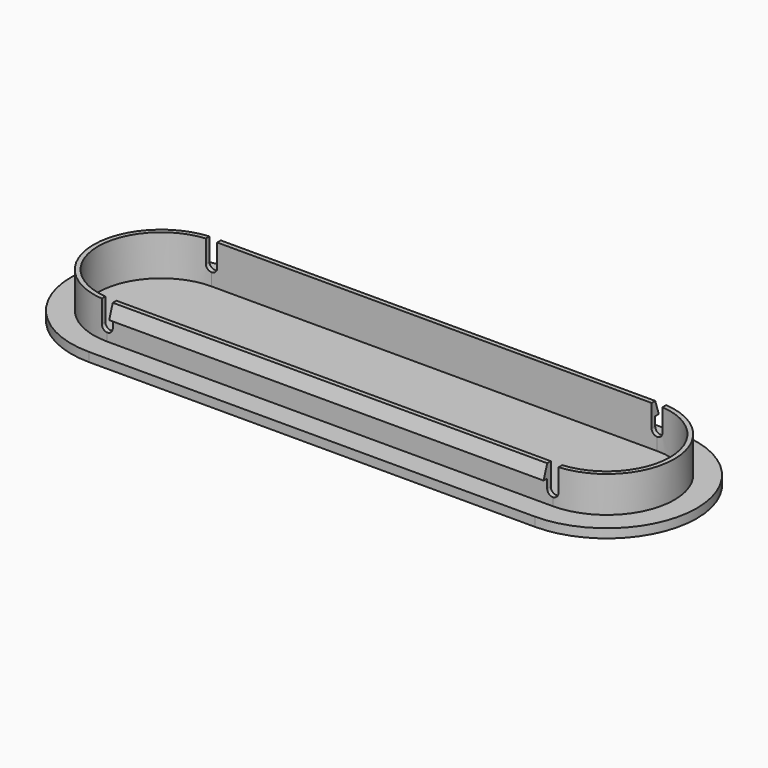
from build123d import *

# Parameters (mm, degrees)
F1_DEPTH      = 2
F2_DEPTH      = 8
F3_T          = 1
F3_T3_DEPTH   = 101
F3_T6_ANGLE   = 180.000000001
F3_T8_ANGLE   = 180.000000001
F7_DEPTH      = 25
F7_DEPTH_BACK = 25


# Not quite as in the source:
# - a shell that OpenCascade refuses in one call is made with other operations: the cavity is built on its own and cut out


with BuildPart() as f1:
    # F0 (on Top) → F1 (new body)
    with BuildSketch(Plane.XY):
        with BuildLine():
            Line((0, 19.999999553), (-99, 19.999999553))
            ThreePointArc((-99, 19.999999553), (-118.999999553, 0), (-99, -19.999999553))
            Line((-99, -19.999999553), (0, -19.999999553))
            ThreePointArc((0, -19.999999553), (19.999999553, 0), (0, 19.999999553))
        make_face()
        with BuildLine():
            ThreePointArc((0, 15), (15, 0), (0, -15))
            Line((0, -15), (-99, -15))
            ThreePointArc((-99, -15), (-114, 0), (-99, 15))
            Line((-99, 15), (0, 15))
        make_face(mode=Mode.SUBTRACT)
        with BuildLine():
            Line((-99, -15), (0, -15))
            ThreePointArc((0, -15), (15, 0), (0, 15))
            Line((0, 15), (-99, 15))
            ThreePointArc((-99, 15), (-114, 0), (-99, -15))
        make_face()
    extrude(amount=-F1_DEPTH)

    # F0 (on Top) → F2 (join)
    with BuildSketch(Plane.XY):
        with BuildLine():
            Line((-99, -15), (0, -15))
            ThreePointArc((0, -15), (15, 0), (0, 15))
            Line((0, 15), (-99, 15))
            ThreePointArc((-99, 15), (-114, 0), (-99, -15))
        make_face()
    extrude(amount=F2_DEPTH)

    # F3: shell of thickness 1, made by hand


with BuildPart() as f3_core1:
    # F3_t2: copy of F1
    add(f1.part)

    # the walls: a layer under each face that stays
    f3_faces = [f3_core1.faces().sort_by_distance(p)[0] for p in [
        (-49.5, -19.999999553, -1),
        (-118.999999553, 0, -1),
        (19.999999553, 0, -1),
        (-109.0714281883, -17.1428567597, 0),
        (-49.5, 0, -2),
        (-49.5, 19.999999553, -1),
        (-49.5, -15, 4),
        (15, 0, 4),
        (-49.5, 15, 4),
        (-114, 0, 4),
    ]]
    thicken(f3_faces, amount=-F3_T, mode=Mode.SUBTRACT)

    # F3_s4 → F3_t3 (cut)
    with BuildSketch(Plane.YZ.offset(-100)):
        Polygon((-15.01, 0.01), (-15, -1), (-14, -1), (-14, 0), align=None)
        Polygon((15.01, 0.01), (15, -1), (14, -1), (14, 0), align=None)
    extrude(amount=F3_T3_DEPTH, mode=Mode.SUBTRACT)

    # F3_s5 → F3_t6 (revolve, cut)
    with BuildSketch(Plane.YZ):
        Polygon((-15.01, 0.01), (-15, -1), (-14, -1), (-14, 0), align=None)
    revolve(axis=Axis((0, 0, 0), (0, 0, 1)), revolution_arc=F3_T6_ANGLE, mode=Mode.SUBTRACT)

    # F3_s7 → F3_t8 (revolve, cut)
    with BuildSketch(Plane.YZ.offset(-99)):
        Polygon((15.01, 0.01), (15, -1), (14, -1), (14, 0), align=None)
    revolve(axis=Axis((-99, 0, 0), (0, 0, 1)), revolution_arc=F3_T8_ANGLE, mode=Mode.SUBTRACT)


with BuildPart() as f1_1:
    add(f1.part)

    # what is left inside the walls is the cavity
    f3_cavity = [f3_core1.part.solids().sort_by_distance(p)[0] for p in [
        (-49.5, -4.666667, 7.99),
    ]]
    add(f3_cavity, mode=Mode.SUBTRACT)

    # F5: sweep along a path in F5_path
    with BuildLine(Plane(origin=(0, 15, 8), x_dir=(0, -1, 0), z_dir=(0, 0, -1))) as f5_path:
        Line((0, 0), (0, 99))
    # F4 (on Right) → F5 (sweep)
    with BuildSketch(Plane.YZ):
        Polygon((16, 5.01), (15, 8), (15, 5.01), align=None)
        Polygon((-15, 5.01), (-15, 8), (-16, 5.01), align=None)
    sweep(path=f5_path.line)

    # F6 (on Front) → F7 (cut, two sides)
    with BuildSketch(Plane.XZ) as f7_sk:
        with BuildLine():
            ThreePointArc((-100.2408070591, 3.0141202733), (-99.000737071, 1.7740502852), (-97.760667083, 3.0141202733))
            Line((-97.760667083, 3.0141202733), (-97.760667083, 9.1903032735))
            Line((-97.760667083, 9.1903032735), (-100.2408070591, 9.8686125129))
            Line((-100.2408070591, 9.8686125129), (-100.2408070591, 3.0141202733))
        make_face()
        with BuildLine():
            Line((-1.2400699881, 9.1903032735), (-1.2400699881, 3.0141202733))
            ThreePointArc((-1.2400699881, 3.0141202733), (0, 1.7740502852), (1.2400699881, 3.0141202733))
            Line((1.2400699881, 3.0141202733), (1.2400699881, 9.8686125129))
            Line((1.2400699881, 9.8686125129), (-1.2400699881, 9.1903032735))
        make_face()
    extrude(amount=-F7_DEPTH, mode=Mode.SUBTRACT)
    extrude(f7_sk.sketch, amount=F7_DEPTH_BACK, mode=Mode.SUBTRACT)


solid = f1_1.part
